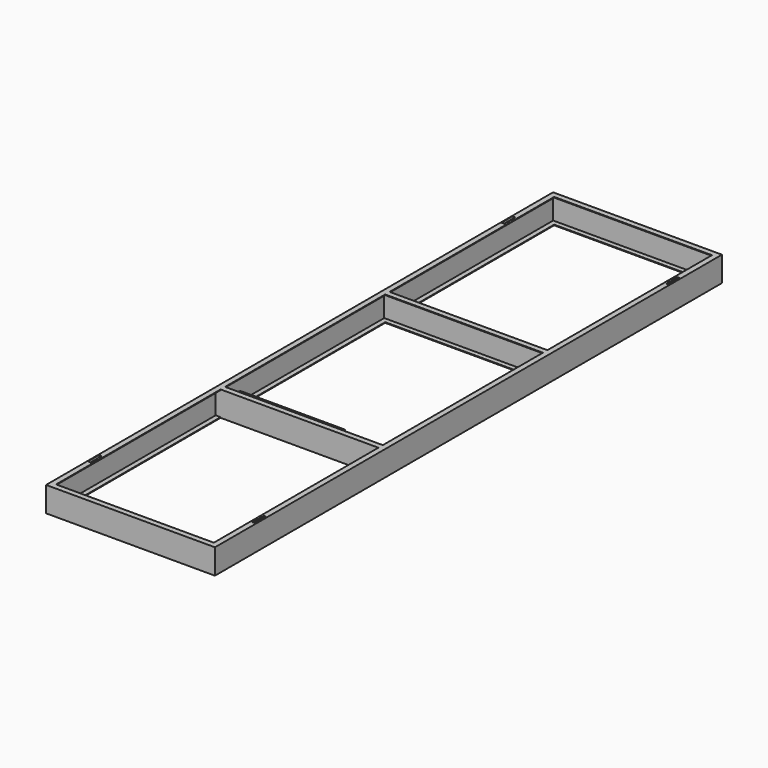
from build123d import *

# Parameters (mm, degrees)
F2_DEPTH  = 11582.4
F6_DEPTH  = 3086.1
F10_W     = 50.8
F10_H     = 254
F11_DEPTH = 11.43
F13_DEPTH = 1930.4


# Not quite as in the source:
# - a pattern or mirror of a feature is missing from the dataset's text; its kind, count and spacing are read off the source's solid


with BuildPart() as f2:
    # F1 (on Front) → F2 (new body, through all)
    with BuildSketch(Plane.XZ):
        Polygon((0, 457.2), (0, 0), (101.6, 0), (101.6, 11.43), (11.43, 11.43), (11.43, 445.77), (101.6, 445.77), (101.6, 457.2), align=None)
    extrude(amount=-F2_DEPTH)

    # F5 (on Right) → F6 (join, through all)
    with BuildSketch(Plane.YZ):
        Polygon((0, 457.2), (0, 0), (101.6, 0), (101.6, 11.43), (11.43, 11.43), (11.43, 445.77), (101.6, 445.77), (101.6, 457.2), align=None)
        Polygon((3860.8, 457.2), (3860.8, 0), (3962.4, 0), (3962.4, 11.43), (3872.23, 11.43), (3872.23, 445.77), (3962.4, 445.77), (3962.4, 457.2), align=None)
    f6 = extrude(amount=F6_DEPTH)

    # F6_copies: F6 across plane
    add(f6.mirror(Plane.ZX.offset(5791.2)))

    # F7: F2 across plane


with BuildPart() as f2_1:
    add(f2.part)
    add(f2.part.mirror(Plane.YZ.offset(1543.05)))

    # F10 (on face) → F11 (cut, through all)
    with BuildSketch(Plane.XY.offset(457.2)):
        with Locations((36.83, 1066.8)):
            Rectangle(F10_W, F10_H)
        with Locations((3049.27, 1066.8)):
            Rectangle(F10_W, F10_H)
    f11 = extrude(amount=-F11_DEPTH, mode=Mode.SUBTRACT)

    # F11_copies: F11 across plane
    add(f11.mirror(Plane.ZX.offset(5791.2)), mode=Mode.SUBTRACT)

    # F12 (on Right) → F13 (join)
    with BuildSketch(Plane.YZ):
        Polygon((4343.4, 177.8), (4343.4, 0), (4419.6, 0), (4419.6, 9.525), (4352.925, 9.525), (4352.925, 168.275), (4419.6, 168.275), (4419.6, 177.8), align=None)
    extrude(amount=F13_DEPTH)


solid = f2_1.part
